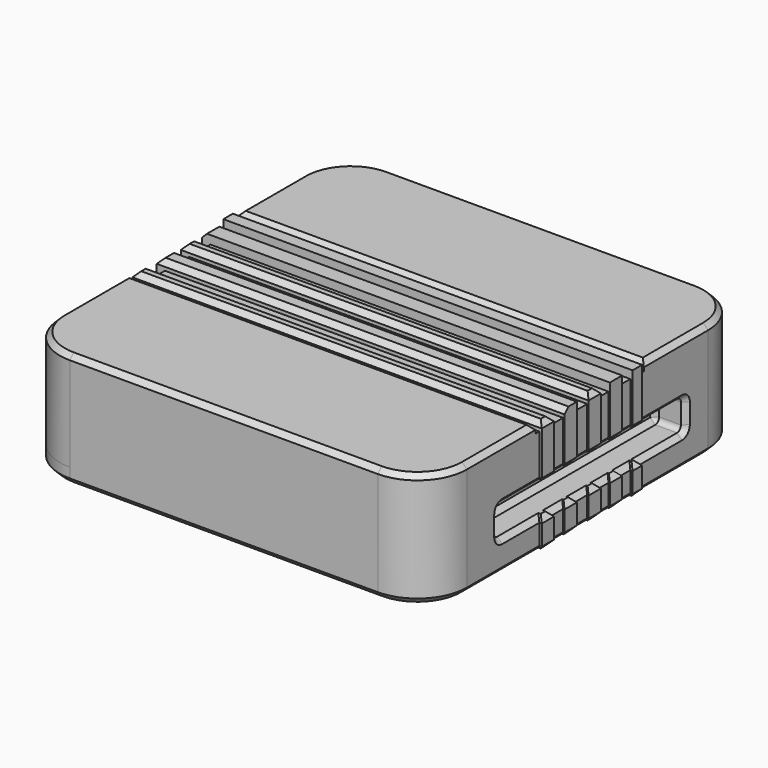
from build123d import *

# Parameters (mm, degrees)
F0_W           = 104.385972023
F0_H           = 102.7361825109
F1_DEPTH       = 25.4
F2_R           = 12.7
F3_W           = 104.385972023
F3_H           = 34.7953215241
F4_DEPTH       = 2.151042223
F5_W           = 34.6233174205
F5_H           = 23.248957777
F6_DEPTH       = 2.2678324021
F7_W           = 105.0066649914
F7_H           = 3.9484277368
F7_W_2         = 104.5954488218
F7_W_3         = 104.9624271691
F7_H_2         = 3.0627343804
F8_DEPTH       = 25.4
F9_SIZE        = 1.27
F11_DEPTH      = 18.542
F11_DEPTH_BACK = 8.128
F12_SIZE       = 1.26999
F13_DEPTH      = 4.064
F14_SIZE       = 1.524


# Not quite as in the source:
# - a fillet or chamfer is up to 0.001 mm smaller than in the source, because OpenCascade refuses the exact size
# - a feature names something its author has since deleted; it is built from what else it names


with BuildPart() as f1:
    # F0 (on Top) → F1 (new body)
    with BuildSketch(Plane.XY):
        with Locations((1.49012e-05, 0.9748823941)):
            Rectangle(F0_W, F0_H)
    extrude(amount=F1_DEPTH)

    # F2
    f2_edges = [f1.edges().sort_by_distance(p)[0] for p in [
        (-52.192971, -50.393209, 12.7),
        (52.193001, -50.393209, 12.7),
        (-52.192971, 52.342974, 12.7),
        (52.193001, 52.342974, 12.7),
    ]]
    fillet(f2_edges, radius=F2_R)

    # F3 (on face) → F4 (cut)
    with BuildSketch(Plane.XY.offset(25.4)):
        with Locations((1.49012e-05, 1.6497857869)):
            Rectangle(F3_W, F3_H)
    extrude(amount=-F4_DEPTH, mode=Mode.SUBTRACT)

    # F5 (on face) → F6 (cut)
    with BuildSketch(Plane(origin=(-52.1929711103, 0, 0), x_dir=(0, -1, 0), z_dir=(-1, 0, 0))):
        with Locations((-1.7357878387, 11.6244788885)):
            Rectangle(F5_W, F5_H)
    extrude(amount=-F6_DEPTH, mode=Mode.SUBTRACT)

    # F7 (on face) → F8 (join)
    with BuildSketch(Plane.XY.offset(25.4)):
        with Locations((0.3103613853, -12.4907959253)):
            Rectangle(F7_W, F7_H)
        with Locations((0.2631898969, -4.8708016984)):
            Rectangle(F7_W_2, F7_H)
        with Locations((0.2631917596, 2.8477641754)):
            Rectangle(F7_W_2, F7_H)
        with Locations((0.2340506762, 9.6958940849)):
            Rectangle(F7_W_2, F7_H)
        with Locations((0.2882424742, 16.2318507209)):
            Rectangle(F7_W_3, F7_H_2)
    extrude(amount=-F8_DEPTH)

    # F9
    f9_edges = [f1.edges().sort_by_distance(p)[0] for p in [
        (-52.192971, 29.34521, 25.4),
        (-48.473227, 48.62323, 25.4),
        (48.473257, 48.62323, 25.4),
        (52.193001, 29.34521, 25.4),
        (1.5e-05, 19.047447, 25.4),
        (1.5e-05, 52.342974, 25.4),
        (0.310361, -10.516582, 25.4),
        (-52.192971, -12.490796, 25.4),
        (0.310361, -14.46501, 25.4),
        (52.813694, -12.490796, 25.4),
        (0.26319, -6.845016, 25.4),
        (0.263192, 4.821978, 25.4),
        (-52.034533, 2.847764, 25.4),
        (0.263192, 0.87355, 25.4),
        (52.560916, 2.847764, 25.4),
        (-52.063674, 9.695894, 25.4),
        (-52.034535, -4.870802, 25.4),
        (52.193001, -26.720542, 25.4),
        (48.473257, -46.673465, 25.4),
        (1.5e-05, -50.393209, 25.4),
        (-48.473227, -46.673465, 25.4),
        (-52.192971, -26.720542, 25.4),
        (1.5e-05, -15.747875, 25.4),
    ]]
    chamfer(f9_edges, length=F9_SIZE)

    # F10 (on face) → F11 (cut, two sides)
    with BuildSketch(Plane.YZ.offset(52.1930009127)) as f11_sk:
        with BuildLine():
            Line((31.2485084504, 11.6244788885), (-26.3840258121, 11.6244788885))
            ThreePointArc((-26.3840258121, 11.6244788885), (-27.2820514243, 11.2525045006), (-27.6540258121, 10.3544788885))
            Line((-27.6540258121, 10.3544788885), (-27.6540258121, 5.2147726174))
            ThreePointArc((-27.6540258121, 5.2147726174), (-27.2820514243, 4.3167470053), (-26.3840258121, 3.9447726174))
            Line((-26.3840258121, 3.9447726174), (31.2485084504, 3.9447726174))
            ThreePointArc((31.2485084504, 3.9447726174), (32.1465340625, 4.3167470053), (32.5185084504, 5.2147726174))
            Line((32.5185084504, 5.2147726174), (32.5185084504, 10.3544788885))
            ThreePointArc((32.5185084504, 10.3544788885), (32.1465340625, 11.2525045006), (31.2485084504, 11.6244788885))
        make_face()
    extrude(amount=F11_DEPTH, mode=Mode.SUBTRACT)
    extrude(f11_sk.sketch, amount=-F11_DEPTH_BACK, mode=Mode.SUBTRACT)

    # F12 (size 1.27 in the source; OpenCascade refuses exactly that, so slightly less here)
    f12_edges = [f1.edges().sort_by_distance(p)[0] for p in [
        (52.193001, -20.424518, 11.624479),
        (52.193001, 24.505863, 11.624479),
        (52.769456, 16.231851, 3.944773),
        (48.129001, -26.384026, 3.944773),
        (44.065001, 2.432241, 3.944773),
        (48.129001, 31.248508, 3.944773),
        (52.193001, 24.505863, 3.944773),
        (52.481228, 17.763218, 3.944773),
        (52.481228, 14.700484, 3.944773),
        (52.193001, 13.185296, 3.944773),
        (52.362388, 11.670108, 3.944773),
        (52.531775, 9.695894, 3.944773),
        (52.362388, 7.72168, 3.944773),
        (52.193001, 6.271829, 3.944773),
        (52.376959, 4.821978, 3.944773),
        (52.560916, 2.847764, 3.944773),
        (52.376959, 0.87355, 3.944773),
        (52.193001, -1.011519, 3.944773),
        (52.376958, -2.896588, 3.944773),
        (52.560914, -4.870802, 3.944773),
        (52.376958, -6.845016, 3.944773),
        (52.193001, -8.680799, 3.944773),
        (52.503347, -10.516582, 3.944773),
        (52.813694, -12.490796, 3.944773),
        (52.503347, -14.46501, 3.944773),
        (52.193001, -20.424518, 3.944773),
        (48.129001, 31.248508, 11.624479),
        (44.065001, 2.432241, 11.624479),
        (48.129001, -26.384026, 11.624479),
        (52.503347, -14.46501, 11.624479),
        (52.813694, -12.490796, 11.624479),
        (52.503347, -10.516582, 11.624479),
        (52.193001, -8.680799, 11.624479),
        (52.376958, -6.845016, 11.624479),
        (52.560914, -4.870802, 11.624479),
        (52.376958, -2.896588, 11.624479),
        (52.193001, -1.011519, 11.624479),
        (52.376959, 0.87355, 11.624479),
        (52.560916, 2.847764, 11.624479),
        (52.376959, 4.821978, 11.624479),
        (52.193001, 6.271829, 11.624479),
        (52.362388, 7.72168, 11.624479),
        (52.531775, 9.695894, 11.624479),
        (52.362388, 11.670108, 11.624479),
        (52.193001, 13.185296, 11.624479),
        (52.481228, 14.700484, 11.624479),
        (52.769456, 16.231851, 11.624479),
        (52.481228, 17.763218, 11.624479),
    ]]
    chamfer(f12_edges, length=F12_SIZE)

    # F13 (add): a face of the model
    f13_faces = [f1.faces().sort_by_distance(p)[0] for p in [
        (0.2236699974, 0.971664384, 0),
    ]]
    extrude(f13_faces, amount=F13_DEPTH)

    # F14
    f14_edges = [f1.edges().sort_by_distance(p)[0] for p in [
        (48.473257, 48.62323, -4.064),
        (1.5e-05, 52.342974, -4.064),
        (-48.473227, 48.62323, -4.064),
        (-52.192971, 29.34521, -4.064),
        (-51.059055, 19.047447, -4.064),
        (-49.925139, 18.405332, -4.064),
        (-51.059055, 17.763218, -4.064),
        (-52.192971, 16.231851, -4.064),
        (-51.059055, 14.700484, -4.064),
        (-49.925139, 13.185296, -4.064),
        (-50.994406, 11.670108, -4.064),
        (-52.063674, 9.695894, -4.064),
        (-50.994406, 7.72168, -4.064),
        (-49.925139, 6.271829, -4.064),
        (-50.979836, 4.821978, -4.064),
        (-52.034533, 2.847764, -4.064),
        (-50.979836, 0.87355, -4.064),
        (-49.925139, -1.011519, -4.064),
        (-50.979837, -2.896588, -4.064),
        (-52.034535, -4.870802, -4.064),
        (-50.979837, -6.845016, -4.064),
        (-49.925139, -8.680799, -4.064),
        (-51.059055, -10.516582, -4.064),
        (-52.192971, -12.490796, -4.064),
        (-51.059055, -14.46501, -4.064),
        (-49.925139, -15.02044, -4.064),
        (-51.059055, -15.575871, -4.064),
        (-52.192971, -26.63454, -4.064),
        (-48.473227, -46.673465, -4.064),
        (1.5e-05, -50.393209, -4.064),
        (48.473257, -46.673465, -4.064),
        (52.193001, -26.079109, -4.064),
        (52.503347, -14.46501, -4.064),
        (52.813694, -12.490796, -4.064),
        (52.503347, -10.516582, -4.064),
        (52.193001, -8.680799, -4.064),
        (52.376958, -6.845016, -4.064),
        (52.560914, -4.870802, -4.064),
        (52.376958, -2.896588, -4.064),
        (52.193001, -1.011519, -4.064),
        (52.376959, 0.87355, -4.064),
        (52.560916, 2.847764, -4.064),
        (52.376959, 4.821978, -4.064),
        (52.193001, 6.271829, -4.064),
        (52.362388, 7.72168, -4.064),
        (52.531775, 9.695894, -4.064),
        (52.362388, 11.670108, -4.064),
        (52.193001, 13.185296, -4.064),
        (52.481228, 14.700484, -4.064),
        (52.769456, 16.231851, -4.064),
        (52.481228, 17.763218, -4.064),
        (52.193001, 28.703096, -4.064),
    ]]
    chamfer(f14_edges, length=F14_SIZE)


solid = f1.part
